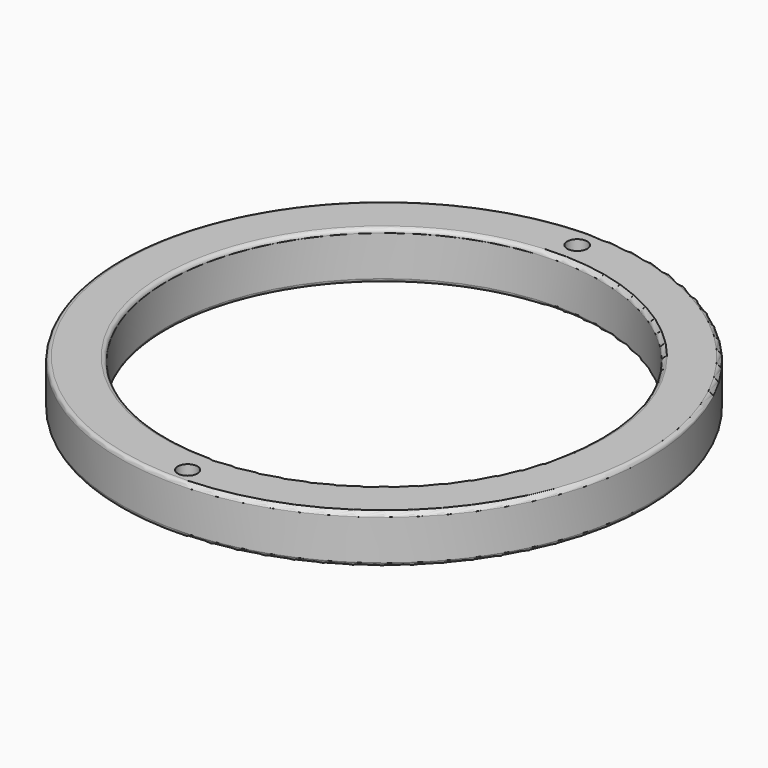
from build123d import *

# Parameters (mm, degrees)
F0_R     = 32.25
F0_R_2   = 1.2
F0_R_3   = 26.5
F0_R_4   = 1.225
F1_DEPTH = 5
F2_DEPTH = 5.9
F3_R     = 0.5
F4_R     = 0.5


with BuildPart() as f1:
    # F0 (on Top) → F1 (new body)
    with BuildSketch(Plane.XY):
        Circle(F0_R)
        with Locations((0, -30)):
            Circle(F0_R_2, mode=Mode.SUBTRACT)
        Circle(F0_R_3, mode=Mode.SUBTRACT)
        with Locations((0, 29.5)):
            Circle(F0_R_4, mode=Mode.SUBTRACT)
    extrude(amount=F1_DEPTH)

    # F0 (on Top) → F2 (join)
    with BuildSketch(Plane.XY):
        Circle(F0_R)
        with Locations((0, -30)):
            Circle(F0_R_2, mode=Mode.SUBTRACT)
        Circle(F0_R_3, mode=Mode.SUBTRACT)
        with Locations((0, 29.5)):
            Circle(F0_R_4, mode=Mode.SUBTRACT)
    extrude(amount=F2_DEPTH)

    # F3
    f3_edges = [f1.edges().sort_by_distance(p)[0] for p in [
        (-26.5, 0, 0),
        (-32.25, 0, 0),
        (-32.25, 0, 5.9),
    ]]
    fillet(f3_edges, radius=F3_R)

    # F4
    f4_edges = [f1.edges().sort_by_distance(p)[0] for p in [
        (-26.5, 0, 5.9),
        (-32.25, 0, 5.4),
    ]]
    fillet(f4_edges, radius=F4_R)


solid = f1.part
